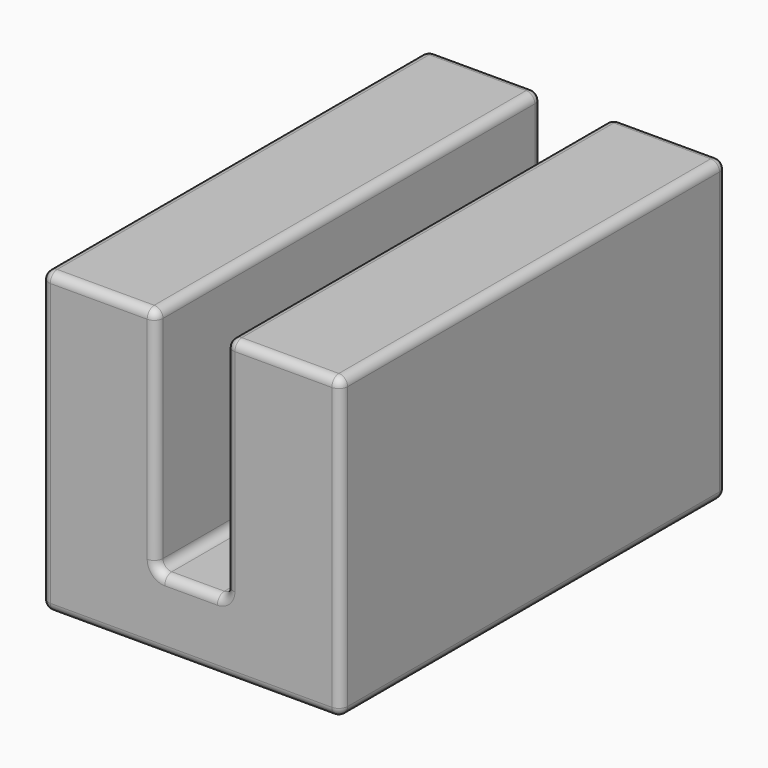
from build123d import *

# Parameters (mm, degrees)
F0_W     = 33.147
F0_H     = 66.294
F1_DEPTH = 69.85
F2_R     = 2.54


with BuildPart() as f1:
    # F0 (on Front) → F1 (new body, symmetric)
    with BuildSketch(Plane.XZ):
        with Locations((-12.4733666049, 21.13100771)):
            Rectangle(F0_W, F0_H)
        Polygon((57.5671333951, -32.33599229), (57.5671333951, -12.01599229), (24.4201333951, -12.01599229), (4.1001333951, -12.01599229), (-29.0468666049, -12.01599229), (-29.0468666049, -32.33599229), align=None)
        with Locations((40.9936333951, 21.13100771)):
            Rectangle(F0_W, F0_H)
    extrude(amount=F1_DEPTH, both=True)

    # F2
    f2_edges = [f1.edges().sort_by_distance(p)[0] for p in [
        (-12.473367, 69.85, 54.278008),
        (-29.046867, 0, 54.278008),
        (-12.473367, -69.85, 54.278008),
        (4.100133, 0, 54.278008),
        (57.567133, 0, 54.278008),
        (40.993633, 69.85, 54.278008),
        (24.420133, 0, 54.278008),
        (40.993633, -69.85, 54.278008),
        (57.567133, 0, -32.335992),
        (57.567133, 69.85, 10.971008),
        (57.567133, -69.85, 10.971008),
        (24.420133, 0, -12.015992),
        (14.260133, 69.85, -12.015992),
        (4.100133, 0, -12.015992),
        (14.260133, -69.85, -12.015992),
        (4.100133, 69.85, 21.131008),
        (4.100133, -69.85, 21.131008),
        (-29.046867, 0, -32.335992),
        (14.260133, 69.85, -32.335992),
        (14.260133, -69.85, -32.335992),
        (-29.046867, 69.85, 10.971008),
        (-29.046867, -69.85, 10.971008),
        (24.420133, 69.85, 21.131008),
        (24.420133, -69.85, 21.131008),
    ]]
    fillet(f2_edges, radius=F2_R)


solid = f1.part
